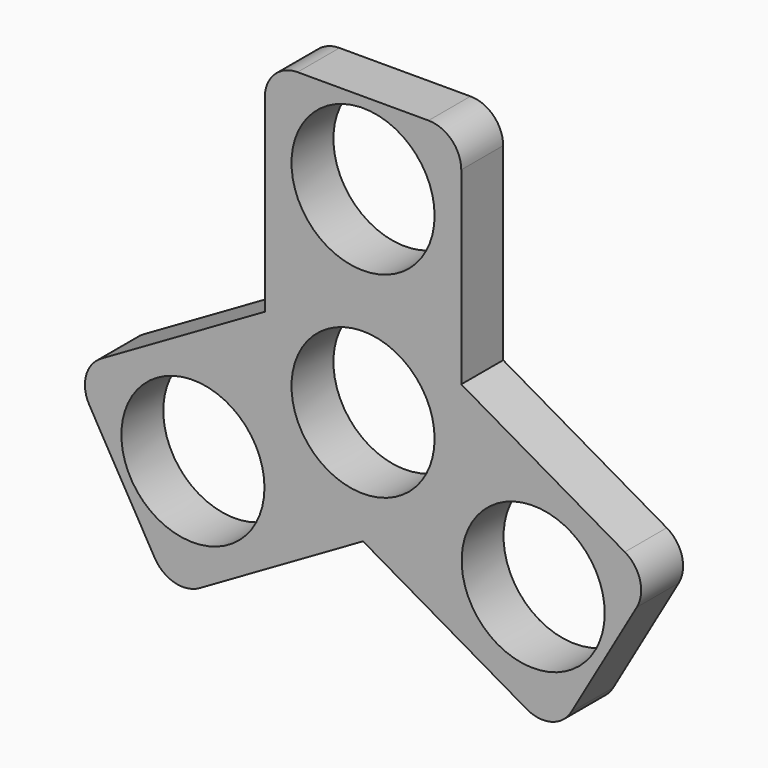
from build123d import *

# Parameters (mm, degrees)
F0_R     = 10.925
F1_DEPTH = 8


with BuildPart() as f1:
    # F0 (on Front) → F1 (new body)
    with BuildSketch(Plane.XZ):
        with BuildLine():
            Line((-225.7977879047, -8.6602540378), (-225.7977879047, -12.5))
            Line((-225.7977879047, -12.5), (-232.4484229994, -12.5))
            Line((-232.4484229994, -12.5), (-240.7977879047, -17.3205080757))
            Line((-240.7977879047, -17.3205080757), (-215.8218352628, -31.7403810568))
            ThreePointArc((-215.8218352628, -31.7403810568), (-212.0277400373, -32.2398831693), (-208.9917082439, -29.9102540378))
            Line((-208.9917082439, -29.9102540378), (-198.9917082439, -12.5897459622))
            ThreePointArc((-198.9917082439, -12.5897459622), (-198.4922061314, -8.7956507366), (-200.8218352628, -5.7596189432))
            Line((-200.8218352628, -5.7596189432), (-225.7977879047, 8.6602540378))
            Line((-225.7977879047, 8.6602540378), (-225.7977879047, -0.9807621135))
            Line((-225.7977879047, -0.9807621135), (-222.4724703574, -6.7403810568))
            Line((-222.4724703574, -6.7403810568), (-225.7977879047, -8.6602540378))
        make_face()
        with Locations((-214.8170257912, -15)):
            Circle(F0_R, mode=Mode.SUBTRACT)
        Polygon((-240.7977879047, -17.3205080757), (-232.4484229994, -12.5), (-249.1471528101, -12.5), align=None)
        with BuildLine():
            Line((-240.7977879047, -17.3205080757), (-249.1471528101, -12.5))
            Line((-249.1471528101, -12.5), (-255.7977879047, -12.5))
            Line((-255.7977879047, -12.5), (-255.7977879047, -8.6602540378))
            Line((-255.7977879047, -8.6602540378), (-259.123105452, -6.7403810568))
            Line((-259.123105452, -6.7403810568), (-255.7977879047, -0.9807621135))
            Line((-255.7977879047, -0.9807621135), (-255.7977879047, 8.6602540378))
            Line((-255.7977879047, 8.6602540378), (-280.7737405467, -5.7596189432))
            ThreePointArc((-280.7737405467, -5.7596189432), (-283.1033696781, -8.7956507366), (-282.6038675656, -12.5897459622))
            Line((-282.6038675656, -12.5897459622), (-272.6038675656, -29.9102540378))
            ThreePointArc((-272.6038675656, -29.9102540378), (-269.5678357722, -32.2398831693), (-265.7737405467, -31.7403810568))
            Line((-265.7737405467, -31.7403810568), (-240.7977879047, -17.3205080757))
        make_face()
        with Locations((-266.7785500183, -15)):
            Circle(F0_R, mode=Mode.SUBTRACT)
        Polygon((-234.1471528101, 13.4807621135), (-225.7977879047, -0.9807621135), (-225.7977879047, 8.6602540378), align=None)
        with BuildLine():
            Line((-234.1471528101, 13.4807621135), (-225.7977879047, 8.6602540378))
            Line((-225.7977879047, 8.6602540378), (-225.7977879047, 37.5))
            ThreePointArc((-225.7977879047, 37.5), (-227.2622539988, 41.0355339059), (-230.7977879047, 42.5))
            Line((-230.7977879047, 42.5), (-250.7977879047, 42.5))
            ThreePointArc((-250.7977879047, 42.5), (-254.3333218107, 41.0355339059), (-255.7977879047, 37.5))
            Line((-255.7977879047, 37.5), (-255.7977879047, 8.6602540378))
            Line((-255.7977879047, 8.6602540378), (-247.4484229994, 13.4807621135))
            Line((-247.4484229994, 13.4807621135), (-244.123105452, 19.2403810568))
            Line((-244.123105452, 19.2403810568), (-240.7977879047, 17.3205080757))
            Line((-240.7977879047, 17.3205080757), (-237.4724703574, 19.2403810568))
            Line((-237.4724703574, 19.2403810568), (-234.1471528101, 13.4807621135))
        make_face()
        with Locations((-240.7977879047, 30)):
            Circle(F0_R, mode=Mode.SUBTRACT)
        Polygon((-255.7977879047, 8.6602540378), (-255.7977879047, -0.9807621135), (-247.4484229994, 13.4807621135), align=None)
        Polygon((-247.4484229994, 13.4807621135), (-240.7977879047, 17.3205080757), (-244.123105452, 19.2403810568), align=None)
        Polygon((-240.7977879047, 17.3205080757), (-234.1471528101, 13.4807621135), (-237.4724703574, 19.2403810568), align=None)
        Polygon((-249.1471528101, -12.5), (-232.4484229994, -12.5), (-225.7977879047, -8.6602540378), (-225.7977879047, -0.9807621135), (-234.1471528101, 13.4807621135), (-240.7977879047, 17.3205080757), (-247.4484229994, 13.4807621135), (-255.7977879047, -0.9807621135), (-255.7977879047, -8.6602540378), align=None)
        with Locations((-240.7977879047, 0)):
            Circle(F0_R, mode=Mode.SUBTRACT)
        Polygon((-225.7977879047, -0.9807621135), (-225.7977879047, -8.6602540378), (-222.4724703574, -6.7403810568), align=None)
        Polygon((-232.4484229994, -12.5), (-225.7977879047, -12.5), (-225.7977879047, -8.6602540378), align=None)
        Polygon((-255.7977879047, -12.5), (-249.1471528101, -12.5), (-255.7977879047, -8.6602540378), align=None)
        Polygon((-259.123105452, -6.7403810568), (-255.7977879047, -8.6602540378), (-255.7977879047, -0.9807621135), align=None)
    extrude(amount=F1_DEPTH)


solid = f1.part
